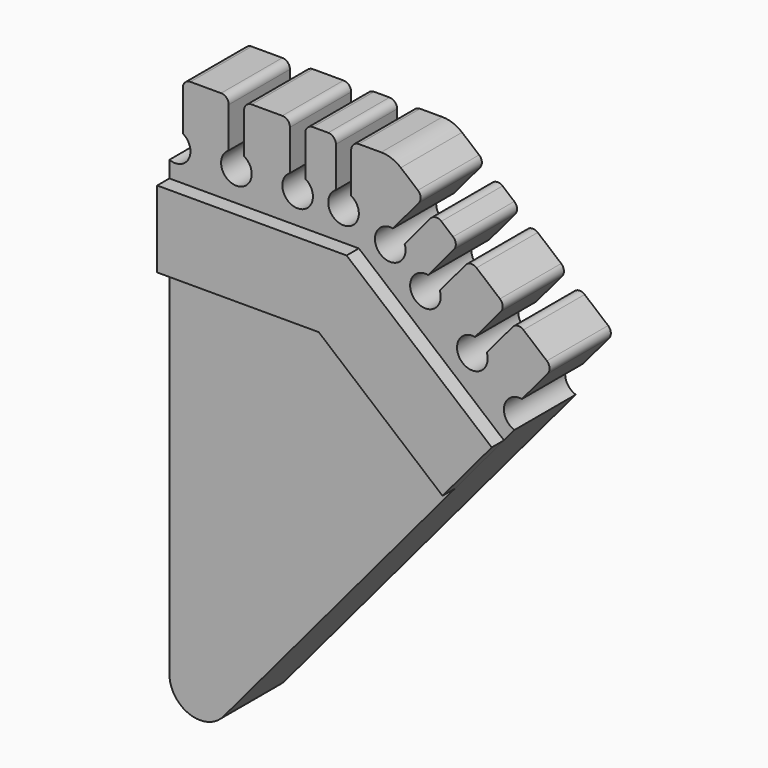
from build123d import *

# Parameters (mm, degrees)
F2_DEPTH = 5
F3_DEPTH = 1
F4_DEPTH = 5
F5_R     = 0.5
F8_R     = 2


with BuildPart() as f2:
    # F0 (on Front) → F2 (new body)
    with BuildSketch(Plane.XZ):
        Polygon((0, 29), (0, 0), (10.5551367937, 29), align=None)
        Polygon((0, 34), (0, 29), (10.5551367937, 29), (12.3749879651, 34), align=None)
        Polygon((12.3749879651, 34), (14.5588093706, 40), (0, 40), (0, 34), align=None)
    extrude(amount=-F2_DEPTH)

    # F1 (on Front) → F4 (cut, through all)
    with BuildSketch(Plane.XZ):
        with BuildLine():
            ThreePointArc((-0.1250120349, 36.8660254038), (-0.1250120349, 35.1339745962), (1.3749879651, 36))
            ThreePointArc((1.3749879651, 36), (1.2410133688, 36.5), (0.8749879651, 36.8660254038))
            ThreePointArc((0.8749879651, 36.8660254038), (0.3749879651, 37), (-0.1250120349, 36.8660254038))
        make_face()
        with BuildLine():
            ThreePointArc((-0.1250120349, 36.8660254038), (0.3749879651, 37), (0.8749879651, 36.8660254038))
            Line((0.8749879651, 36.8660254038), (0.8749879651, 40))
            Line((0.8749879651, 40), (-0.1250120349, 40))
            Line((-0.1250120349, 40), (-0.1250120349, 36.8660254038))
        make_face()
        with BuildLine():
            ThreePointArc((3.8749879651, 36.8660254038), (3.8749879651, 35.1339745962), (5.3749879651, 36))
            ThreePointArc((5.3749879651, 36), (5.2410133688, 36.5), (4.8749879651, 36.8660254038))
            ThreePointArc((4.8749879651, 36.8660254038), (4.3749879651, 37), (3.8749879651, 36.8660254038))
        make_face()
        with BuildLine():
            ThreePointArc((3.8749879651, 36.8660254038), (4.3749879651, 37), (4.8749879651, 36.8660254038))
            Line((4.8749879651, 36.8660254038), (4.8749879651, 40))
            Line((4.8749879651, 40), (3.8749879651, 40))
            Line((3.8749879651, 40), (3.8749879651, 36.8660254038))
        make_face()
        with BuildLine():
            ThreePointArc((10.8749879651, 36.8660254038), (10.8749879651, 35.1339745962), (12.3749879651, 36))
            ThreePointArc((12.3749879651, 36), (12.2410133688, 36.5), (11.8749879651, 36.8660254038))
            ThreePointArc((11.8749879651, 36.8660254038), (11.3749879651, 37), (10.8749879651, 36.8660254038))
        make_face()
        with BuildLine():
            ThreePointArc((7.8749879651, 36.8660254038), (7.8749879651, 35.1339745962), (9.3749879651, 36))
            ThreePointArc((9.3749879651, 36), (9.2410133688, 36.5), (8.8749879651, 36.8660254038))
            ThreePointArc((8.8749879651, 36.8660254038), (8.3749879651, 37), (7.8749879651, 36.8660254038))
        make_face()
        with BuildLine():
            ThreePointArc((7.8749879651, 36.8660254038), (8.3749879651, 37), (8.8749879651, 36.8660254038))
            Line((8.8749879651, 36.8660254038), (8.8749879651, 40))
            Line((8.8749879651, 40), (7.8749879651, 40))
            Line((7.8749879651, 40), (7.8749879651, 36.8660254038))
        make_face()
        with BuildLine():
            ThreePointArc((10.8749879651, 36.8660254038), (11.3749879651, 37), (11.8749879651, 36.8660254038))
            Line((11.8749879651, 36.8660254038), (11.8749879651, 40))
            Line((11.8749879651, 40), (10.8749879651, 40))
            Line((10.8749879651, 40), (10.8749879651, 36.8660254038))
        make_face()
    extrude(amount=-F4_DEPTH, mode=Mode.SUBTRACT)

    # F5
    f5_edges = [f2.edges().sort_by_distance(p)[0] for p in [
        (0.874988, 2.5, 40),
        (3.874988, 2.5, 40),
        (4.874988, 2.5, 40),
        (11.874988, 2.5, 40),
        (10.874988, 2.5, 40),
        (7.874988, 2.5, 40),
        (8.874988, 2.5, 40),
    ]]
    fillet(f5_edges, radius=F5_R)

    # F6: F2 across face


with BuildPart() as f3:
    # F0 (on Front) → F3 (new body)
    with BuildSketch(Plane.XZ):
        Polygon((0, 34), (0, 29), (10.5551367937, 29), (12.3749879651, 34), align=None)
    extrude(amount=F3_DEPTH)

    # F7: F3 across face


with BuildPart() as f2_1:
    add(f2.part)
    add(f2.part.mirror(Plane(origin=(7.2794046853, 2.5, 20), x_dir=(0, 1, 0), z_dir=(0.9396926208, 0, -0.3420201433))))

    # F8
    f8_edges = [f2_1.edges().sort_by_distance(p)[0] for p in [
        (14.558809, 2.5, 40),
        (0, 2.5, 0),
    ]]
    fillet(f8_edges, radius=F8_R)


with BuildPart() as f3_1:
    add(f3.part)
    add(f3.part.mirror(Plane(origin=(11.4650623794, -0.5, 31.5), x_dir=(0, 1, 0), z_dir=(0.9396926208, 0, -0.3420201433))))


solid = Compound([f2_1.part, f3_1.part])
